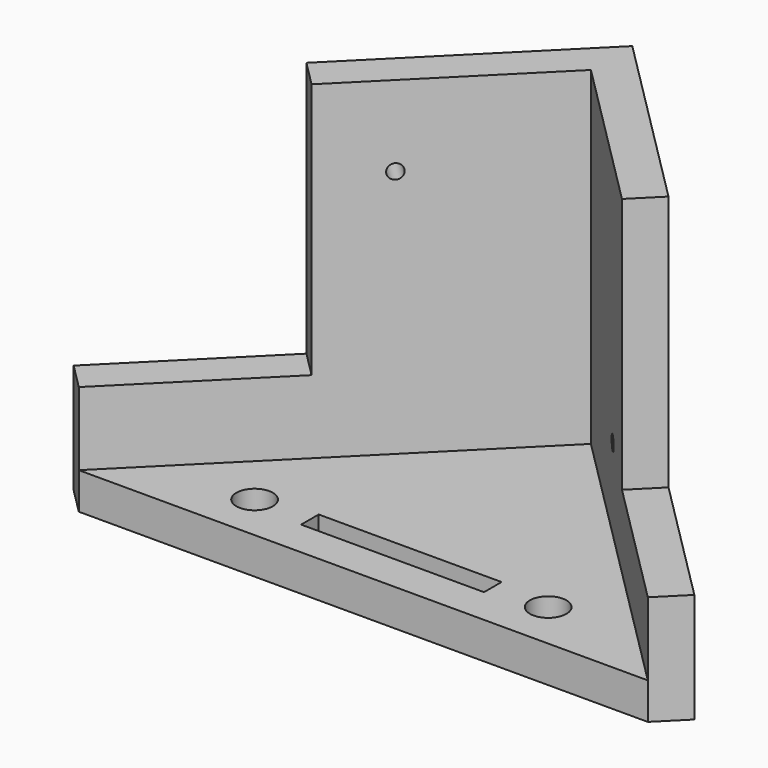
from build123d import *

# Parameters (mm, degrees)
F1_DEPTH  = 50
F3_DEPTH  = 5
F4_W      = 25
F4_H      = 3
F4_R      = 2.5
F5_DEPTH  = 25
F6_R      = 1
F8_DEPTH  = 25
F7_R      = 1
F9_DEPTH  = 25
F13_DEPTH = 35


# Not quite as in the source:
# - a feature names something its author has since deleted; it is built from what else it names


with BuildPart() as f1:
    # F0 (on Top) → F1 (new body)
    with BuildSketch(Plane.XY):
        Polygon((0, 42.4264068712), (-42.4264068712, 0), (-38.8908729653, -3.5355339059), (0, 35.3553390593), (38.8908729653, -3.5355339059), (42.4264068712, 0), align=None)
    extrude(amount=F1_DEPTH)

    # F2 (on face) → F3 (join)
    with BuildSketch(Plane(origin=(0, 0, 0), x_dir=(1, 0, 0), z_dir=(0, 0, -1))):
        Polygon((38.8908729653, 3.5355339059), (-38.8908729653, 3.5355339059), (0, -35.3553390593), align=None)
    extrude(amount=-F3_DEPTH)

    # F4 (on face) → F5 (cut)
    with BuildSketch(Plane(origin=(0, 0, 0), x_dir=(1, 0, 0), z_dir=(0, 0, -1))):
        with Locations((0, -2.9644660941)):
            Rectangle(F4_W, F4_H)
        with Locations((20, -3.0505650211)):
            Circle(F4_R)
        with Locations((-20, -2.8942257773)):
            Circle(F4_R)
    extrude(amount=-F5_DEPTH, mode=Mode.SUBTRACT)

    # F6 (on face) → F8 (cut)
    with BuildSketch(Plane(origin=(-17.6776695297, 17.6776695297, 0), x_dir=(0.7071067812, 0.7071067812, 0), z_dir=(0.7071067812, -0.7071067812, 0))):
        with Locations((4, 39)):
            Circle(F6_R)
    extrude(amount=-F8_DEPTH, mode=Mode.SUBTRACT)

    # F7 (on face) → F9 (cut)
    with BuildSketch(Plane(origin=(17.6776695297, 17.6776695297, 0), x_dir=(0.7071067812, -0.7071067812, 0), z_dir=(-0.7071067812, -0.7071067812, 0))):
        with Locations((-4, 16)):
            Circle(F7_R)
    extrude(amount=-F9_DEPTH, mode=Mode.SUBTRACT)

    # F12 (on face) → F13 (cut)
    with BuildSketch(Plane.XY.offset(50)):
        Polygon((-38.8908729653, -3.5355339059), (-21.2132034356, 14.1421356237), (-24.7487373415, 17.6776695297), (-42.4264068712, 0), align=None)
        Polygon((24.7487373415, 17.6776695297), (21.2132034356, 14.1421356237), (38.8908729653, -3.5355339059), (42.4264068712, 0), align=None)
    extrude(amount=-F13_DEPTH, mode=Mode.SUBTRACT)


solid = f1.part
